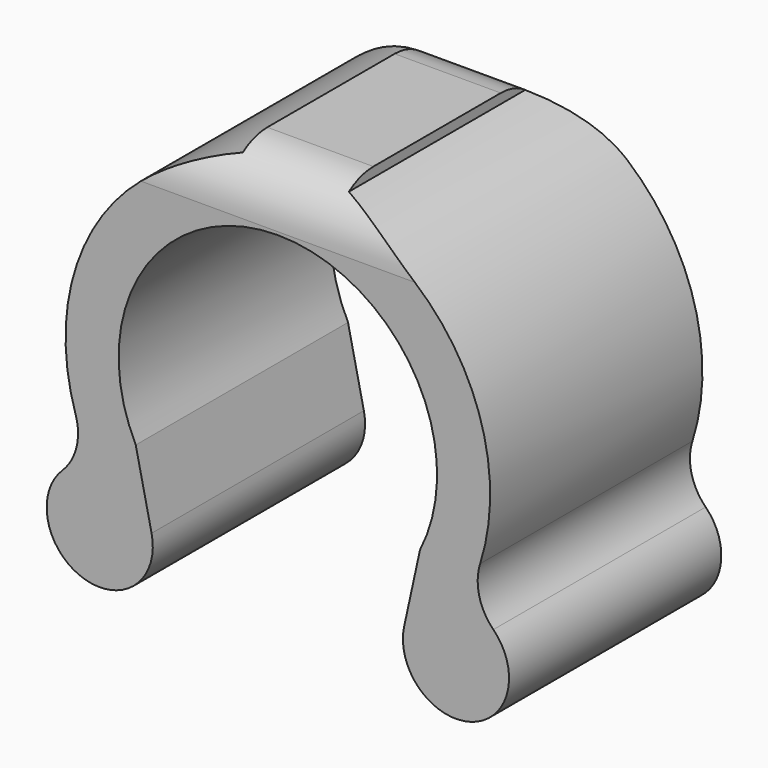
from build123d import *

# Parameters (mm, degrees)
F1_DEPTH = 25
F3_R     = 5


# Not quite as in the source:
# - a feature names something its author has since deleted; it is built from what else it names


with BuildPart() as f1:
    # F0 (on Front) → F1 (new body)
    with BuildSketch(Plane.XZ):
        with BuildLine():
            ThreePointArc((11.8972236274, -13.5987717306), (19.6369586065, -18.770230883), (17.4821764595, -9.7146027319))
            ThreePointArc((17.4821764595, -9.7146027319), (18.3784296837, 7.8888099459), (5, 19.364916731))
            Line((5, 19.364916731), (5, 20.2805753797))
            Line((5, 20.2805753797), (0, 20.2805753797))
            Line((0, 20.2805753797), (0, 20))
            Line((0, 20), (0, 15))
            ThreePointArc((0, 15), (12.7749432268, 7.86135011), (13.3904401788, -6.7598899265))
            Line((13.3904401788, -6.7598899265), (11.8972236274, -13.5987717306))
        make_face()
    extrude(amount=F1_DEPTH)

    # F2: F1 across plane


with BuildPart() as f1_1:
    add(f1.part)
    add(f1.part.mirror(Plane.YZ))

    # F3
    f3_edges = [f1_1.edges().sort_by_distance(p)[0] for p in [
        (-17.482176, -12.5, -9.714603),
        (17.482176, -12.5, -9.714603),
        (0, -25, 20.280575),
        (0, 0, 20.280575),
    ]]
    fillet(f3_edges, radius=F3_R)


solid = f1_1.part
